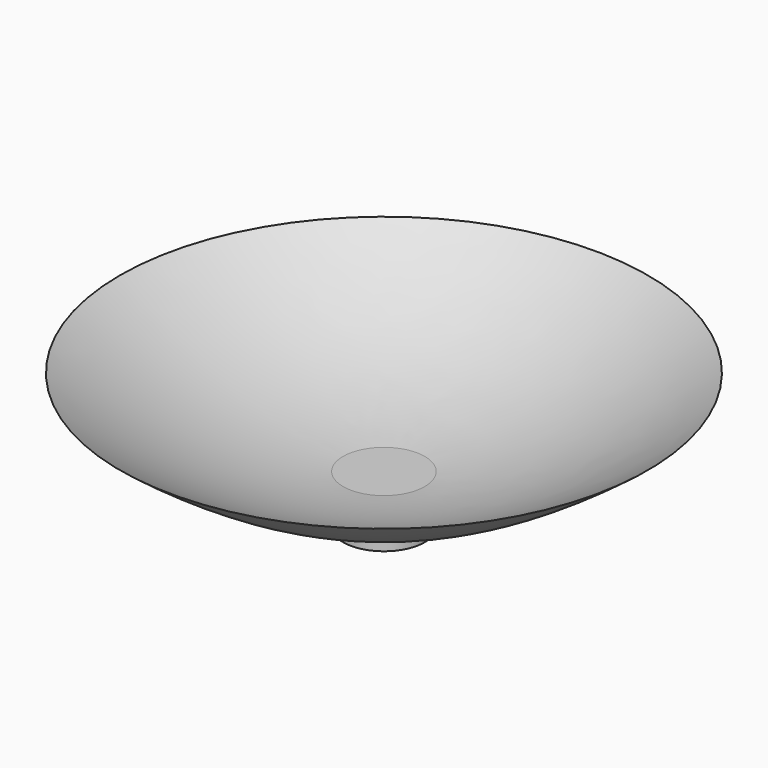
from build123d import *

# Parameters (mm, degrees)
F3_R     = 1.25
F4_DEPTH = 37.2983106457
F5_R     = 0.1


with BuildPart() as f1:
    # F0 (on Front) → F1 (revolve)
    with BuildSketch(Plane.XZ):
        with BuildLine():
            add(Edge.make_bspline(
                [(-5, 4.0937988318), (-7.4889216128, 4.4831718575), (-12.2515039896, 5.551606316), (-19.0092734521, 8.1400270742), (-25.568362861, 11.7589006204), (-30.0299528469, 14.8981568753), (-32.2973105457, 16.6326323425)],
                knots=[0.0002435476, 0.0002435476, 0.0002435476, 0.0002435476, 0.25, 0.5, 0.75, 0.9911285082, 0.9911285082, 0.9911285082, 0.9911285082], degree=3))
            Line((-5, 4.0937988318), (-5, 6))
            add(Edge.make_bspline(
                [(-5, 6), (-14.7075803578, 7.0438257777), (-22.3108520529, 10.0535693462), (-32.2973105457, 16.6326323425)],
                knots=[0, 0, 0, 0, 29.2949830783, 29.2949830783, 29.2949830783, 29.2949830783], degree=3))
        make_face()
        Polygon((-5, 0), (0, 0), (0, 6), (-5, 6), (-5, 4.0937988318), align=None)
    revolve(axis=Axis((0, 0, 3), (0, 0, -1)))

    # F3 (on line) → F4 (cut, through all)
    with BuildSketch(Plane.YZ.offset(-5)):
        with Locations((-0.0001267018, 2.2674880456)):
            Circle(F3_R)
    extrude(amount=F4_DEPTH, mode=Mode.SUBTRACT)

    # F5
    f5_edges = [f1.edges().sort_by_distance(p)[0] for p in [
        (-4.921263, 0.883839, 3.151289),
        (-4.921263, 0.883839, 1.383687),
        (-4.841196, -1.250127, 2.267488),
        (4.841196, -1.250127, 2.267488),
    ]]
    fillet(f5_edges, radius=F5_R)


solid = f1.part
